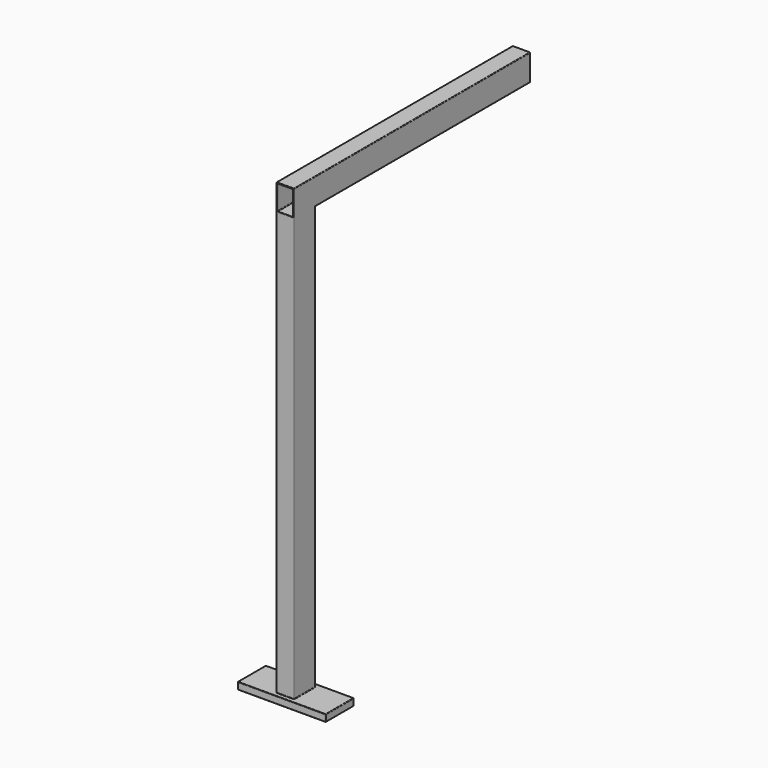
from build123d import *

# Parameters (mm, degrees)
F0_W     = 250
F0_H     = 100
F1_DEPTH = 20
F2_W     = 50
F2_H     = 75
F2_W_2   = 44
F2_H_2   = 69
F3_DEPTH = 1200
F4_W     = 50
F4_H     = 75
F4_W_2   = 44
F4_H_2   = 69
F5_DEPTH = 837.2
F6_F1_R  = 1.5
F6_F2_R  = 1.5
F6_F3_R  = 1.5
F6_F4_R  = 1.4999


# Not quite as in the source:
# - a fillet or chamfer is up to 0.001 mm smaller than in the source, because OpenCascade refuses the exact size


with BuildPart() as f1:
    # F0 (on Top) → F1 (new body)
    with BuildSketch(Plane.XY):
        Rectangle(F0_W, F0_H)
    extrude(amount=F1_DEPTH)

    # F2 (on face) → F3 (join)
    with BuildSketch(Plane.XY.offset(20)):
        Rectangle(F2_W, F2_H)
        Rectangle(F2_W_2, F2_H_2, mode=Mode.SUBTRACT)
    extrude(amount=F3_DEPTH)

    # F4 (on face) → F5 (join)
    with BuildSketch(Plane.XZ.offset(37.5)):
        with Locations((0, 1257.5)):
            Rectangle(F4_W, F4_H)
        with Locations((0, 1257.5)):
            Rectangle(F4_W_2, F4_H_2, mode=Mode.SUBTRACT)
    extrude(amount=-F5_DEPTH)

    # F6: fillet of radius 1.5 on 44 edges, made by hand

    # F6_f1
    f6_f1_edges = [f1.edges().sort_by_distance(p)[0] for p in [
        (-22, -34.5, 620),
        (22, 34.5, 620),
        (22, -34.5, 620),
        (-22, 34.5, 620),
        (-22, 381.1, 1292),
        (22, 381.1, 1292),
        (0, 37.5, 1220),
        (22, 381.1, 1223),
        (-22, 381.1, 1223),
        (22, 0, 1220),
        (0, -34.5, 1220),
        (-22, 0, 1220),
        (0, 34.5, 1220),
        (0, 34.5, 20),
        (-22, 0, 20),
        (22, 0, 20),
        (0, -34.5, 20),
    ]]
    fillet(f6_f1_edges, radius=F6_F1_R)

    # F6_f2
    f6_f2_edges = [f1.edges().sort_by_distance(p)[0] for p in [
        (-25, -37.5, 657.5),
        (25, 37.5, 619.25),
        (25, -37.5, 657.5),
        (-25, 37.5, 619.25),
        (25, 381.1, 1295),
        (-25, 381.1, 1295),
        (0, -37.5, 1295),
        (125, -50, 10),
        (-125, -50, 10),
        (125, 50, 10),
        (0, -50, 0),
        (0, -50, 20),
        (0, 50, 20),
        (125, 0, 20),
        (-125, 0, 20),
        (-125, 50, 10),
        (0, 50, 0),
        (125, 0, 0),
        (-125, 0, 0),
        (-25, 37.9393398282, 1219.5606601718),
        (25, 37.9393398282, 1219.5606601718),
    ]]
    fillet(f6_f2_edges, radius=F6_F2_R)

    # F6_f3
    f6_f3_edges = [f1.edges().sort_by_distance(p)[0] for p in [
        (25, 0, 20),
        (-25, 0, 20),
        (0, -37.5, 20),
        (0, 37.5, 20),
        (24.5606601718, 37.0606601718, 20),
        (-24.5606601718, 37.0606601718, 20),
        (-24.5606601718, -37.0606601718, 20),
        (24.5606601718, -37.0606601718, 20),
    ]]
    fillet(f6_f3_edges, radius=F6_F3_R)

    # F6_f4 (radius 1.5 in the source; OpenCascade refuses exactly that, so slightly less here)
    f6_f4_edges = [f1.edges().sort_by_distance(p)[0] for p in [
        (-22, -37.5, 1257.5),
        (0, -37.5, 1223),
        (0, -37.5, 1292),
        (22, -37.5, 1257.5),
        (21.5606601718, -37.5, 1291.5606601718),
        (21.5606601718, -37.5, 1223.4393398282),
        (-21.5606601718, -37.5, 1291.5606601718),
        (-21.5606601718, -37.5, 1223.4393398282),
    ]]
    fillet(f6_f4_edges, radius=F6_F4_R)


solid = f1.part
